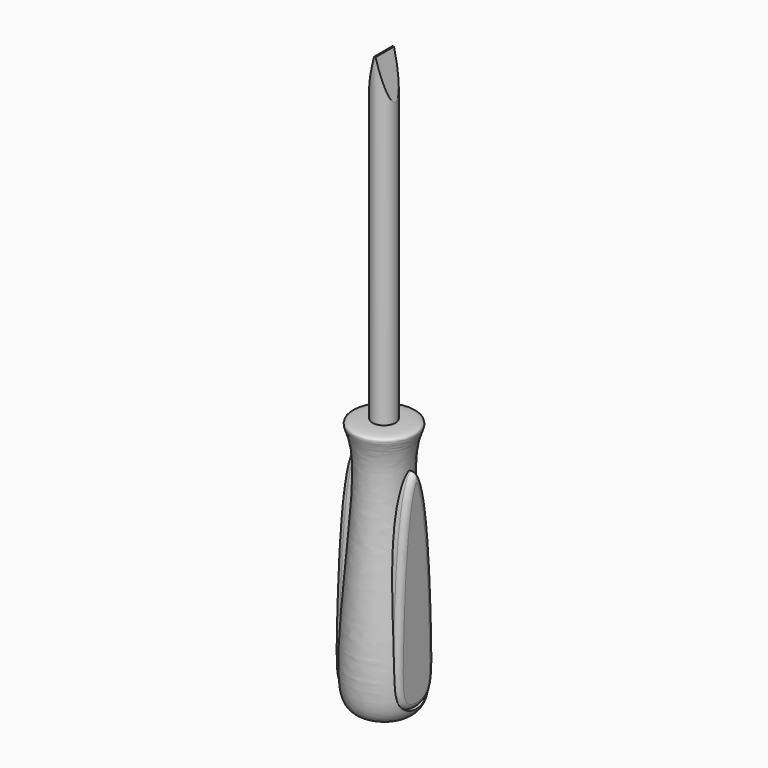
from build123d import *

# Parameters (mm, degrees)
F3_R     = 3.175
F4_DEPTH = 88.9
F6_DEPTH = 12.7
F8_DEPTH = 11.26037
F9_DEPTH = 8.93399
F10_R    = 1.524


with BuildPart() as f1:
    # F0 (on Front) → F1 (revolve)
    with BuildSketch(Plane.XZ):
        with BuildLine():
            Line((0, 27.9473034515), (0, -43.1167059937))
            add(Edge.make_bspline(
                [(0, -43.1167059937), (7.4437569243, -43.1167059937), (12.8562285582, -37.91779643), (4.4967931515, 17.932435438), (9.4614541481, 27.338063369), (8.3568424187, 27.9473034515), (0, 27.9473034515)],
                knots=[0, 0, 0, 0, 0.2093909405, 0.6518504897, 0.8222856605, 1, 1, 1, 1], degree=3))
        make_face()
    revolve(axis=Axis((0, 0, -6.6679045558), (0, 0, -1)))

    # F7 (on Right) → F8 (cut, symmetric)
    with BuildSketch(Plane.YZ):
        with BuildLine():
            add(Edge.make_bspline(
                [(0, 17.6920224884), (4.526096173, 15.8164318834), (6.2397766621, -24.9779351034), (6.22830825, -38.1574120531), (1.4100619542, -39.4739153343), (0, -39.4739153343)],
                knots=[0, 0, 0, 0, 0.5235709405, 0.8273883175, 1, 1, 1, 1], degree=3))
            add(Edge.make_bspline(
                [(0, 17.6920224884), (-4.526096173, 15.8164318834), (-6.2397766621, -24.9779351034), (-6.22830825, -38.1574120531), (-1.4100619542, -39.4739153343), (0, -39.4739153343)],
                knots=[0, 0, 0, 0, 0.5235709405, 0.8273883175, 1, 1, 1, 1], degree=3))
        make_face()
    extrude(amount=F8_DEPTH, both=True, mode=Mode.SUBTRACT)


with BuildPart() as f4:
    # F3 (on face) → F4 (new body)
    with BuildSketch(Plane.XY.offset(27.9473034515)):
        Circle(F3_R)
    extrude(amount=F4_DEPTH)

    # F5 (on Front) → F6 (cut, symmetric)
    with BuildSketch(Plane.XZ):
        Polygon((-3.5795057588, 104.1473034515), (-0.2117474651, 116.8473034515), (-3.5795057588, 116.8473034515), align=None)
        Polygon((3.5795057588, 104.1473034515), (3.5795057588, 116.8473034515), (0.2117474651, 116.8473034515), align=None)
    extrude(amount=F6_DEPTH, both=True, mode=Mode.SUBTRACT)


with BuildPart() as f9:
    # F7 (on Right) → F9 (new body, symmetric)
    with BuildSketch(Plane.YZ):
        with BuildLine():
            add(Edge.make_bspline(
                [(0, 17.6920224884), (4.526096173, 15.8164318834), (6.2397766621, -24.9779351034), (6.22830825, -38.1574120531), (1.4100619542, -39.4739153343), (0, -39.4739153343)],
                knots=[0, 0, 0, 0, 0.5235709405, 0.8273883175, 1, 1, 1, 1], degree=3))
            add(Edge.make_bspline(
                [(0, 17.6920224884), (-4.526096173, 15.8164318834), (-6.2397766621, -24.9779351034), (-6.22830825, -38.1574120531), (-1.4100619542, -39.4739153343), (0, -39.4739153343)],
                knots=[0, 0, 0, 0, 0.5235709405, 0.8273883175, 1, 1, 1, 1], degree=3))
        make_face()
    extrude(amount=F9_DEPTH, both=True)

    # F10
    f10_edges = [f9.edges().sort_by_distance(p)[0] for p in [
        (8.93399, -5.553926, -12.111011),
        (-8.93399, -5.553926, -12.111011),
        (-8.93399, 5.947197, -21.904459),
        (8.93399, 5.947197, -21.904459),
    ]]
    fillet(f10_edges, radius=F10_R)


solid = Compound([f1.part, f4.part, f9.part])
